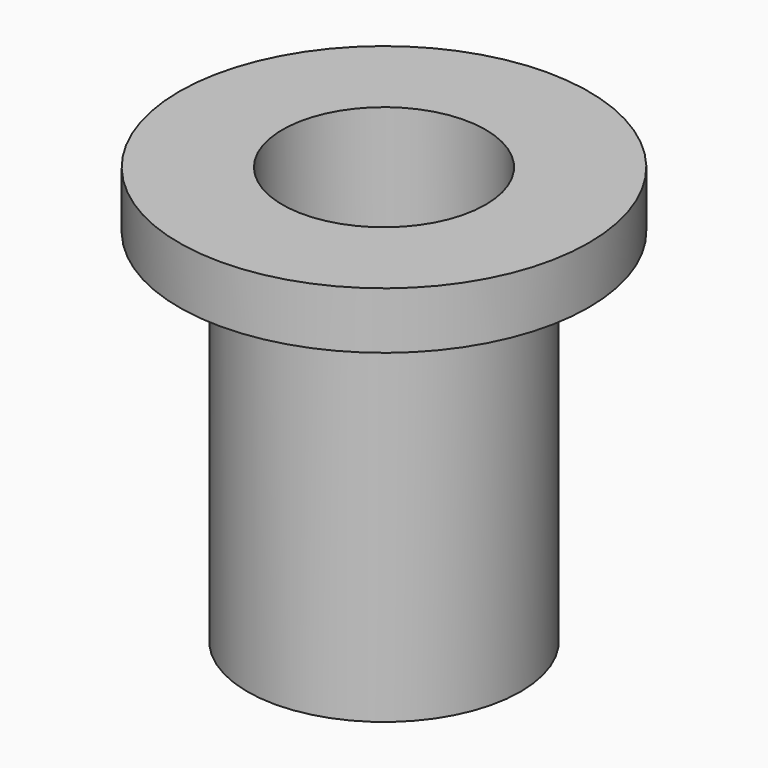
from build123d import *

# Parameters (mm, degrees)
F0_R     = 4.7625
F1_DEPTH = 9.7028
F2_R     = 2.3622
F3_DEPTH = 9.7028
F4_R     = 4.7625
F4_R_2   = 3.175
F5_DEPTH = 8.382


with BuildPart() as f1:
    # F0 (on Top) → F1 (new body)
    with BuildSketch(Plane.XY):
        Circle(F0_R)
    extrude(amount=F1_DEPTH)

    # F2 (on face) → F3 (cut, through all)
    with BuildSketch(Plane.XY.offset(9.7028)):
        Circle(F2_R)
    extrude(amount=-F3_DEPTH, mode=Mode.SUBTRACT)

    # F4 (on face) → F5 (cut)
    with BuildSketch(Plane(origin=(0, 0, 0), x_dir=(1, 0, 0), z_dir=(0, 0, -1))):
        Circle(F4_R)
        Circle(F4_R_2, mode=Mode.SUBTRACT)
    extrude(amount=-F5_DEPTH, mode=Mode.SUBTRACT)


solid = f1.part
